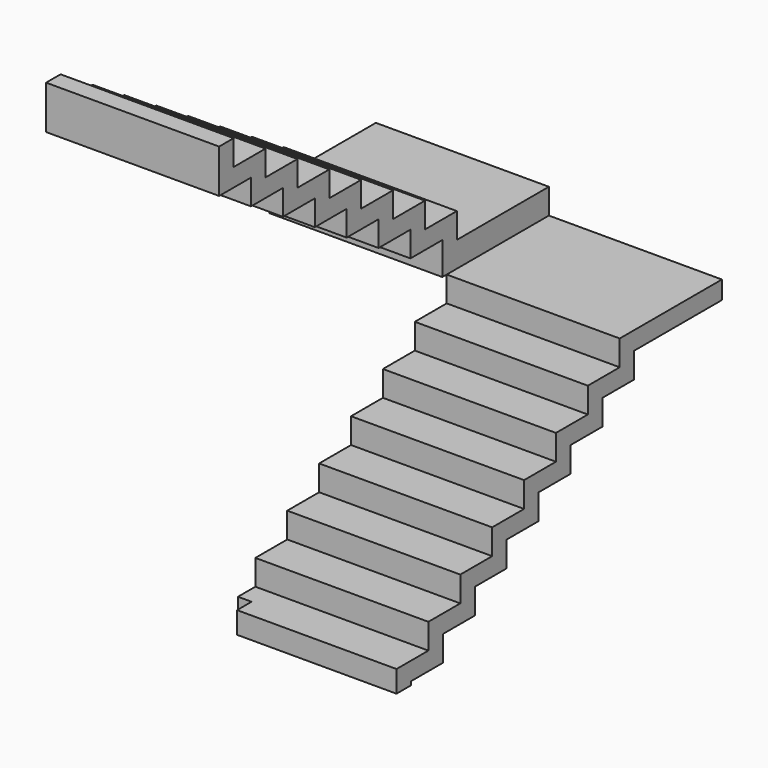
from build123d import *

# Parameters (mm, degrees)
F2_W     = 1117.6
F2_H     = 127
F3_DEPTH = 152.4
F5_DEPTH = 1212.85
F7_DEPTH = 1212.85


# Not quite as in the source:
# - a variable given as a bare number and used for a length is read in inches; the dataset says mm whatever the document's units were


with BuildPart() as f3:
    # F2 (on Top) → F3 (new body)
    with BuildSketch(Plane.XY):
        with Locations((654.05, -1873.25)):
            Rectangle(F2_W, F2_H)
    extrude(amount=F3_DEPTH)

    # F4 (on Right) → F5 (join)
    with BuildSketch(Plane.YZ):
        Polygon((-1657.35, 152.4), (-1809.75, 152.4), (-1809.75, 25.4), (-1530.35, 25.4), (-1530.35, 203.2), (-1250.95, 203.2), (-1250.95, 381), (-971.55, 381), (-971.55, 558.8), (-692.15, 558.8), (-692.15, 736.6), (-412.75, 736.6), (-412.75, 914.4), (-133.35, 914.4), (-133.35, 1092.2), (146.05, 1092.2), (146.05, 1270), (914.4, 1270), (914.4, 1397), (19.05, 1397), (19.05, 1219.2), (-260.35, 1219.2), (-260.35, 1041.4), (-539.75, 1041.4), (-539.75, 863.6), (-819.15, 863.6), (-819.15, 685.8), (-1098.55, 685.8), (-1098.55, 508), (-1377.95, 508), (-1377.95, 330.2), (-1657.35, 330.2), align=None)
    extrude(amount=F5_DEPTH)


with BuildPart() as f7:
    # F6 (on Right) → F7 (new body)
    with BuildSketch(Plane.YZ):
        Polygon((-19.05, 1397), (914.4, 1397), (914.4, 1574.8), (107.95, 1574.8), (107.95, 1752.6), (-171.45, 1752.6), (-171.45, 1930.4), (-450.85, 1930.4), (-450.85, 2108.2), (-730.25, 2108.2), (-730.25, 2286), (-1009.65, 2286), (-1009.65, 2463.8), (-1289.05, 2463.8), (-1289.05, 2641.6), (-1568.45, 2641.6), (-1568.45, 2819.4), (-1847.85, 2819.4), (-1847.85, 2997.2), (-1974.85, 2997.2), (-1974.85, 2692.4), (-1695.45, 2692.4), (-1695.45, 2514.6), (-1416.05, 2514.6), (-1416.05, 2336.8), (-1136.65, 2336.8), (-1136.65, 2159), (-857.25, 2159), (-857.25, 1981.2), (-577.85, 1981.2), (-577.85, 1803.4), (-298.45, 1803.4), (-298.45, 1625.6), (-19.05, 1625.6), align=None)
    extrude(amount=-F7_DEPTH)


solid = Compound([f3.part, f7.part])
